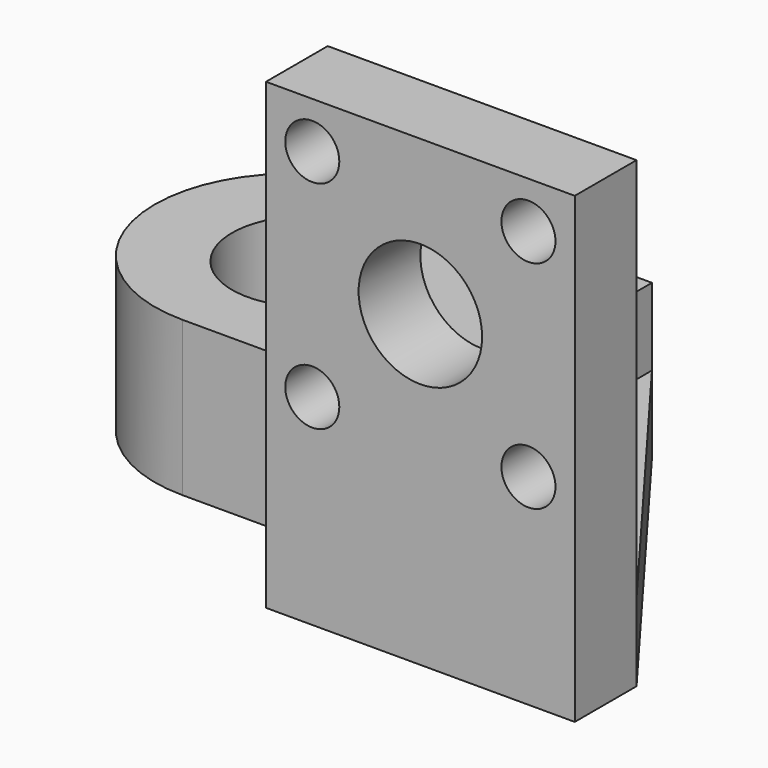
from build123d import *

# Parameters (mm, degrees)
F0_R          = 1.75
F0_R_2        = 4
F0_W          = 5
F0_H          = 10
F1_DEPTH      = 5
F2_DEPTH      = 5
F2_DEPTH_BACK = 20
F3_R          = 5
F4_DEPTH      = 10
F6_DEPTH      = 5


with BuildPart() as f1:
    # F0 (on Front) → F1 (new body)
    with BuildSketch(Plane.XZ):
        Polygon((10, -10), (10, 10), (-10, 10), (-10, -10), (-5, -10), (-5, -20), (5, -20), (5, -10), align=None)
        with Locations((-7, -7)):
            Circle(F0_R, mode=Mode.SUBTRACT)
        with Locations((7, -7)):
            Circle(F0_R, mode=Mode.SUBTRACT)
        with Locations((-7, 7)):
            Circle(F0_R, mode=Mode.SUBTRACT)
        Circle(F0_R_2, mode=Mode.SUBTRACT)
        with Locations((7, 7)):
            Circle(F0_R, mode=Mode.SUBTRACT)
        with Locations((7.5, -15)):
            Rectangle(F0_W, F0_H)
    extrude(amount=F1_DEPTH)

    # F0 (on Front) → F2 (join, two sides)
    with BuildSketch(Plane.XZ) as f2_sk:
        with Locations((-7.5, -15)):
            Rectangle(F0_W, F0_H)
    extrude(amount=F2_DEPTH)
    extrude(f2_sk.sketch, amount=-F2_DEPTH_BACK)

    # F3 (on face) → F4 (join)
    with BuildSketch(Plane(origin=(0, 0, -20), x_dir=(1, 0, 0), z_dir=(0, 0, -1))):
        with BuildLine():
            Line((-21, -20), (-10, -20))
            Line((-10, -20), (-10, -2))
            Line((-10, -2), (-21, -2))
            ThreePointArc((-21, -2), (-27.3639610307, -4.6360389693), (-30, -11))
            ThreePointArc((-30, -11), (-27.3639610307, -17.3639610307), (-21, -20))
        make_face()
        with Locations((-20, -11)):
            Circle(F3_R, mode=Mode.SUBTRACT)
    extrude(amount=-F4_DEPTH)

    # F5 (on face) → F6 (join)
    with BuildSketch(Plane(origin=(0, 0, -20), x_dir=(1, 0, 0), z_dir=(0, 0, -1))):
        Polygon((-10, 5), (-10, 0), (-5, 0), (10, 0), (10, 5), align=None)
        Polygon((10, 0), (-5, 0), (-5, -20), align=None)
    extrude(amount=-F6_DEPTH)


solid = f1.part
